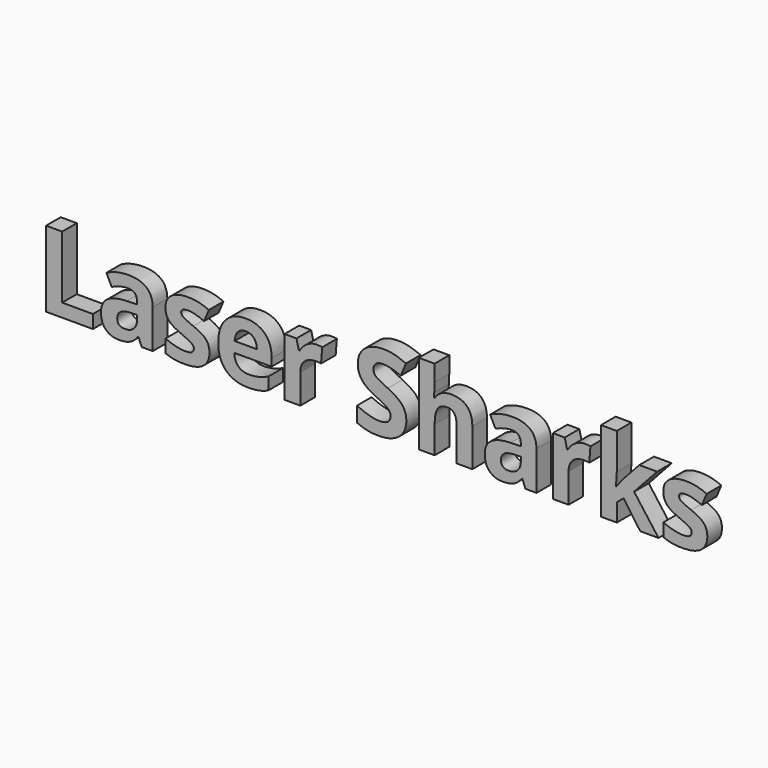
from build123d import *

# Parameters (mm, degrees)
F0_TEXT_SIZE = 156.716783388
F1_DEPTH     = 27


# Not quite as in the source:
# - Text() gives the source's letters only with a copy of the font that has no kerning and outlines rounded to 1/6400 em; it was checked with that copy


with BuildPart() as f1:
    # F0 (on Front) → F1 (new body)
    with BuildSketch(Plane.XZ):
        with Locations((-500.635927824, -51.6670648167)):
            Text('Laser Sharks', F0_TEXT_SIZE, font='Open Sans', font_style=FontStyle.BOLD, text_align=(TextAlign.LEFT, TextAlign.BOTTOM))
    extrude(amount=F1_DEPTH)


solid = f1.part
